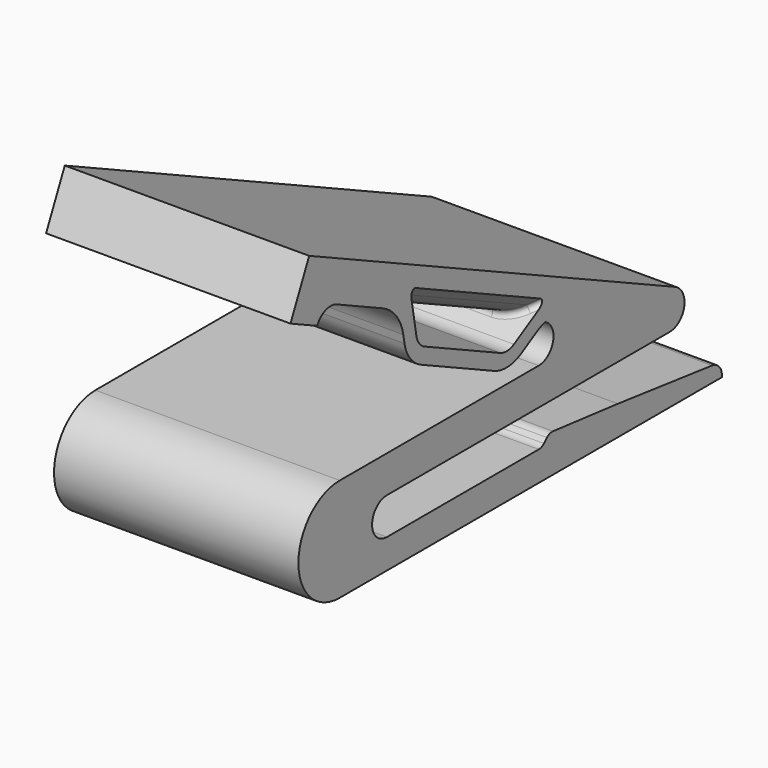
from build123d import *

# Parameters (mm, degrees)
F1_DEPTH    = 13.25
F2_DEPTH    = 13.25
F3_R        = 1
F4_R        = 1.99999
F5_T1_DEPTH = 26.5
F6_R        = 4
F7_SIZE     = 2
F8_R        = 4
F9_R        = 2
F10_R       = 0.5


# Not quite as in the source:
# - a fillet or chamfer that OpenCascade refuses, or shapes differently, is made with other operations: its cross-section is extruded or revolved along the edge and cut away or added
# - a fillet or chamfer is up to 0.001 mm smaller than in the source, because OpenCascade refuses the exact size


with BuildPart() as f1:
    # F0 (on Right) → F1 (new body, symmetric)
    with BuildSketch(Plane.YZ):
        with BuildLine():
            Line((24.5604159161, 8.2188727885), (-25.0402941419, 31.3480637385))
            Line((-25.0402941419, 31.3480637385), (-27.5760037124, 25.9102170163))
            Line((-27.5760037124, 25.9102170163), (-23.9507725642, 24.2197439694))
            Line((-23.9507725642, 24.2197439694), (-23.1055360408, 26.0323595434))
            Line((-23.1055360408, 26.0323595434), (-12.7312477201, 21.1947494516))
            Line((-12.7312477201, 21.1947494516), (-10.9610116945, 20.3692748361))
            Line((-10.9610116945, 20.3692748361), (4.9900053574, 12.9311934295))
            Line((4.9900053574, 12.9311934295), (6.760241383, 12.105718814))
            Line((6.760241383, 12.105718814), (7.7089287185, 11.6633386442))
            Line((7.7089287185, 11.6633386442), (15.0956095835, 8.2188727885))
            Line((15.0956095835, 8.2188727885), (7.7089287185, 8.2188727885))
            Line((7.7089287185, 8.2188727885), (-20.8974118188, 8.2188727885))
            ThreePointArc((-20.8974118188, 8.2188727885), (-26.4974118188, 2.6188727885), (-20.8974118188, -2.9811272115))
            Line((-20.8974118188, -2.9811272115), (30.894998731, -2.9811272115))
            ThreePointArc((30.894998731, -2.9811272115), (30.580160342, -1.8806088655), (29.580710732, -1.3226085804))
            Line((29.580710732, -1.3226085804), (16.8007476451, 0.2188727885))
            Line((16.8007476451, 0.2188727885), (6.4900759503, 0.2188727885))
            Line((6.4900759503, 0.2188727885), (-14.5099240497, 0.2188727885))
            ThreePointArc((-14.5099240497, 0.2188727885), (-16.5099240497, 2.2188727885), (-14.5099240497, 4.2188727885))
            Line((-14.5099240497, 4.2188727885), (24.5604159161, 4.2188727885))
            ThreePointArc((24.5604159161, 4.2188727885), (25.8345564377, 6.2188727885), (24.5604159161, 8.2188727885))
        make_face()
        Polygon((-10.9610116945, 20.3692748361), (-12.7312477201, 21.1947494516), (-11.7561154197, 15.664499365), (1.8970210747, 9.2979372598), (6.760241383, 12.105718814), (4.9900053574, 12.9311934295), (1.8183399389, 11.1000315463), (-10.3250558464, 16.762589997), align=None)
    extrude(amount=F1_DEPTH, both=True)

    # F0 (on Right) → F2 (join, symmetric)
    with BuildSketch(Plane.YZ):
        with BuildLine():
            Line((15.0956095835, 8.2188727885), (7.7089287185, 11.6633386442))
            ThreePointArc((7.7089287185, 11.6633386442), (8.806112099, 9.9411057164), (7.7089287185, 8.2188727885))
            Line((7.7089287185, 8.2188727885), (15.0956095835, 8.2188727885))
        make_face()
        with BuildLine():
            Line((24.5604159161, 8.2188727885), (-25.0402941419, 31.3480637385))
            Line((-25.0402941419, 31.3480637385), (-27.5760037124, 25.9102170163))
            Line((-27.5760037124, 25.9102170163), (-23.9507725642, 24.2197439694))
            Line((-23.9507725642, 24.2197439694), (-23.1055360408, 26.0323595434))
            Line((-23.1055360408, 26.0323595434), (-12.7312477201, 21.1947494516))
            Line((-12.7312477201, 21.1947494516), (-10.9610116945, 20.3692748361))
            Line((-10.9610116945, 20.3692748361), (4.9900053574, 12.9311934295))
            Line((4.9900053574, 12.9311934295), (6.760241383, 12.105718814))
            Line((6.760241383, 12.105718814), (7.7089287185, 11.6633386442))
            Line((7.7089287185, 11.6633386442), (15.0956095835, 8.2188727885))
            Line((15.0956095835, 8.2188727885), (7.7089287185, 8.2188727885))
            Line((7.7089287185, 8.2188727885), (-20.8974118188, 8.2188727885))
            ThreePointArc((-20.8974118188, 8.2188727885), (-26.4974118188, 2.6188727885), (-20.8974118188, -2.9811272115))
            Line((-20.8974118188, -2.9811272115), (30.894998731, -2.9811272115))
            ThreePointArc((30.894998731, -2.9811272115), (30.580160342, -1.8806088655), (29.580710732, -1.3226085804))
            Line((29.580710732, -1.3226085804), (16.8007476451, 0.2188727885))
            Line((16.8007476451, 0.2188727885), (6.4900759503, 0.2188727885))
            Line((6.4900759503, 0.2188727885), (-14.5099240497, 0.2188727885))
            ThreePointArc((-14.5099240497, 0.2188727885), (-16.5099240497, 2.2188727885), (-14.5099240497, 4.2188727885))
            Line((-14.5099240497, 4.2188727885), (24.5604159161, 4.2188727885))
            ThreePointArc((24.5604159161, 4.2188727885), (25.8345564377, 6.2188727885), (24.5604159161, 8.2188727885))
        make_face()
        Polygon((7.5313132472, 1.2188727885), (6.4900759503, 0.2188727885), (16.8007476451, 0.2188727885), align=None)
    extrude(amount=F2_DEPTH, both=True)

    # F3
    f3_edges = [f1.edges().sort_by_distance(p)[0] for p in [
        (0, 6.490076, 0.218873),
        (0, 7.531313, 1.218873),
        (0, 16.800748, 0.218873),
    ]]
    fillet(f3_edges, radius=F3_R)

    # F4 (radius 2 in the source; OpenCascade refuses exactly that, so slightly less here)
    f4_edges = [f1.edges().sort_by_distance(p)[0] for p in [
        (0, -23.105536, 26.03236),
        (0, 24.560416, 8.218873),
        (0, 24.560416, 4.218873),
        (0, 7.708929, 8.218873),
        (0, 7.708929, 11.663339),
    ]]
    fillet(f4_edges, radius=F4_R)

    # F5: fillet of radius 5 on 2 edges, made by hand

    # F5_s2 → F5_t1 (join)
    with BuildSketch(Plane.YZ.offset(-13.25)):
        with BuildLine():
            ThreePointArc((-12.2792701217, 18.6314571149), (-13.2365421853, 20.8070233716), (-15.090217578, 22.2947551617))
            Line((-15.090217578, 22.2947551617), (-12.7312477201, 21.1947494516))
            Line((-12.7312477201, 21.1947494516), (-12.2792701217, 18.6314571149))
        make_face()
        with BuildLine():
            ThreePointArc((6.9194699805, 12.0314692995), (6.3536054599, 11.8292518467), (5.8160865891, 11.5606107896))
            Line((5.8160865891, 11.5606107896), (6.760241383, 12.105718814))
            Line((6.760241383, 12.105718814), (6.9194699805, 12.0314692995))
        make_face()
    extrude(amount=F5_T1_DEPTH)

    # F6
    f6_edges = [f1.edges().sort_by_distance(p)[0] for p in [
        (0, 1.897021, 9.297937),
        (0, -11.756115, 15.664499),
    ]]
    fillet(f6_edges, radius=F6_R)

    # F7
    f7_edges = [f1.edges().sort_by_distance(p)[0] for p in [
        (13.25, -2.985503, 16.650234),
        (-13.25, -2.985503, 16.650234),
    ]]
    chamfer(f7_edges, length=F7_SIZE)

    # F8
    f8_edges = [f1.edges().sort_by_distance(p)[0] for p in [
        (-11.25, -2.985503, 16.650234),
        (11.25, -2.985503, 16.650234),
    ]]
    fillet(f8_edges, radius=F8_R)

    # F9
    f9_edges = [f1.edges().sort_by_distance(p)[0] for p in [
        (0, -10.325056, 16.76259),
        (0, 1.81834, 11.100032),
    ]]
    fillet(f9_edges, radius=F9_R)

    # F10
    f10_edges = [f1.edges().sort_by_distance(p)[0] for p in [
        (-11.167025, 5.331118, 13.128135),
        (-11.167025, -11.029409, 20.757174),
        (11.123879, -11.025557, 20.735332),
        (0, -10.961012, 20.369275),
        (11.123879, 5.31191, 13.117045),
        (0, 4.990005, 12.931193),
    ]]
    fillet(f10_edges, radius=F10_R)


solid = f1.part
